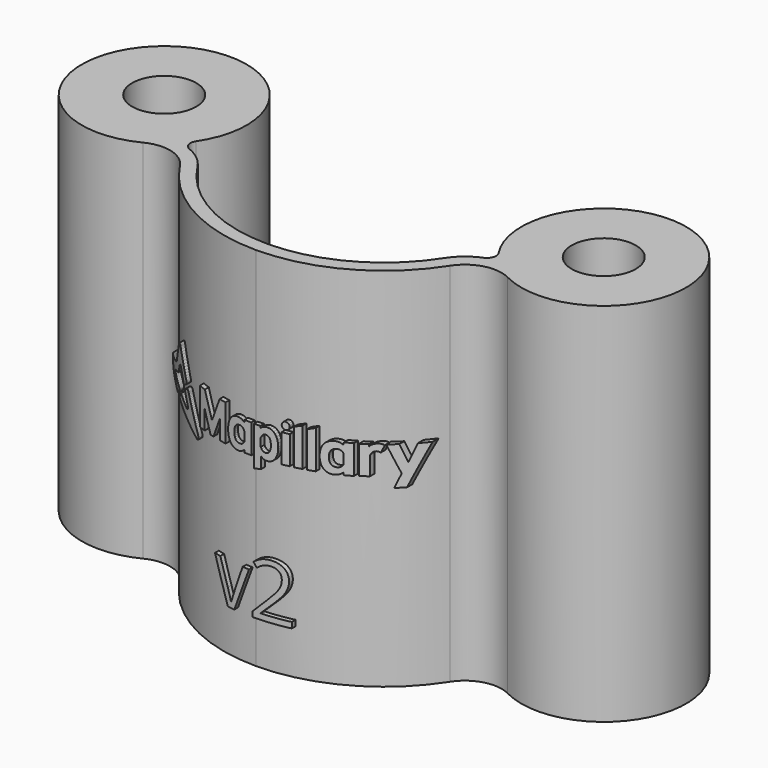
from build123d import *

# Parameters (mm, degrees)
F0_R         = 3.5
F1_DEPTH     = 40
F2_R         = 1
F4_W         = 0.766563
F4_H         = 3.09612
F4_TEXT_SIZE = 8.333333
F5_DEPTH     = 25
F6_W         = 87.868996
F6_H         = 45.529967
F7_DEPTH     = 60


# Not quite as in the source:
# - Text() gives the source's letters only with a copy of the font that has no kerning and outlines rounded to 1/6400 em; it was checked with that copy


with BuildPart() as f1:
    # F0 (on Top) → F1 (new body)
    with BuildSketch(Plane.XY):
        with BuildLine():
            ThreePointArc((-13.476744, -8.624231), (-15.168201, -6.941285), (-17.413215, -6.133047))
            ThreePointArc((-17.413215, -6.133047), (-29.41554, 7.188318), (-19.921875, -8.023023))
            ThreePointArc((-19.921875, -8.023023), (-17.059302, -7.729103), (-14.740189, -9.432753))
            ThreePointArc((-14.740189, -9.432753), (-8.401691, -15.351273), (0, -17.5))
            ThreePointArc((0, -17.5), (8.401691, -15.351273), (14.740189, -9.432753))
            ThreePointArc((14.740189, -9.432753), (17.059302, -7.729103), (19.921875, -8.023023))
            ThreePointArc((19.921875, -8.023023), (29.41554, 7.188318), (17.413215, -6.133047))
            ThreePointArc((17.413215, -6.133047), (15.168201, -6.941285), (13.476744, -8.624231))
            ThreePointArc((13.476744, -8.624231), (7.681546, -14.03545), (0, -16))
            ThreePointArc((0, -16), (-7.681546, -14.03545), (-13.476744, -8.624231))
        make_face()
        with Locations((-24, 0)):
            Circle(F0_R, mode=Mode.SUBTRACT)
        with Locations((24, 0)):
            Circle(F0_R, mode=Mode.SUBTRACT)
    extrude(amount=F1_DEPTH)

    # F2
    f2_edges = [f1.edges().sort_by_distance(p)[0] for p in [
        (-17.413215, -6.133047, 20),
        (17.413215, -6.133047, 20),
    ]]
    fillet(f2_edges, radius=F2_R)

    # F4 (on offset) → F5 (join)
    with BuildSketch(Plane.XZ.offset(25)):
        Polygon((-10.73702, 20.972938), (-10.658014, 20.9132), (-10.637207, 20.902077), (-10.599738, 20.881931), (-10.546861, 20.853384), (-10.479554, 20.816981), (-10.399024, 20.773344), (-10.306352, 20.723018), (-10.202674, 20.666702), (-10.089023, 20.605097), (-9.966599, 20.538592), (-9.836497, 20.467886), (-9.699768, 20.393602), (-9.557594, 20.316362), (-9.411072, 20.236711), (-9.261307, 20.155271), (-9.109379, 20.072742), (-8.956447, 19.989513), (-8.803601, 19.90644), (-8.651977, 19.823911), (-8.502616, 19.742782), (-8.356739, 19.663364), (-8.215367, 19.586436), (-8.079641, 19.512541), (-7.950683, 19.44238), (-7.829612, 19.376419), (-7.717486, 19.315436), (-7.61548, 19.259898), (-7.524667, 19.210505), (-7.446214, 19.167724), (-7.381139, 19.132332), (-7.330665, 19.104719), (-7.29581, 19.085739), (-7.27771, 19.075705), (-7.203309, 19.04887), (-7.131647, 19.048481), (-7.066658, 19.070416), (-7.012178, 19.110786), (-6.972096, 19.165779), (-6.950231, 19.231118), (-6.950519, 19.303302), (-6.976771, 19.377974), (-6.986649, 19.396331), (-7.005551, 19.431957), (-7.032939, 19.483761), (-7.068222, 19.550266), (-7.110754, 19.630539), (-7.159921, 19.723569), (-7.215171, 19.828033), (-7.275851, 19.942765), (-7.341384, 20.066675), (-7.411141, 20.198597), (-7.484577, 20.33752), (-7.561, 20.482042), (-7.639873, 20.631232), (-7.720566, 20.783767), (-7.802473, 20.938713), (-7.884978, 21.094748), (-7.967515, 21.250861), (-8.049469, 21.405729), (-8.130201, 21.558264), (-8.209113, 21.707376), (-8.285621, 21.851899), (-8.359135, 21.990744), (-8.429071, 22.122666), (-8.494728, 22.246576), (-8.55554, 22.36123), (-8.611, 22.465538), (-8.66037, 22.55849), (-8.703073, 22.638763), (-8.738566, 22.705191), (-8.766249, 22.75684), (-8.785408, 22.792231), (-8.795535, 22.810511), (-8.852722, 22.874605), (-8.930203, 22.913886), (-9.016878, 22.922131), (-9.101491, 22.89304), (-9.181671, 22.843491), (-9.261346, 22.795032), (-9.33405, 22.75225), (-9.393306, 22.719581), (-9.473525, 22.659998), (-9.512899, 22.589293), (-9.515396, 22.509719), (-9.484882, 22.423301), (-9.45656, 22.368697), (-9.422468, 22.303203), (-9.383599, 22.229074), (-9.340849, 22.147945), (-9.295236, 22.061605), (-9.24771, 21.97192), (-9.199313, 21.880679), (-9.150908, 21.789672), (-9.103514, 21.700764), (-9.058064, 21.615902), (-9.015571, 21.536562), (-8.977006, 21.464845), (-8.943317, 21.402384), (-8.915471, 21.351202), (-8.894414, 21.312855), (-8.881121, 21.289286), (-8.857778, 21.223714), (-8.860314, 21.159465), (-8.884116, 21.100115), (-8.924455, 21.049322), (-8.976702, 21.010819), (-9.036207, 20.987951), (-9.098193, 20.984606), (-9.158079, 21.004285), (-9.180746, 21.016808), (-9.222562, 21.039755), (-9.280877, 21.071491), (-9.352913, 21.110694), (-9.435932, 21.155731), (-9.527251, 21.205357), (-9.624061, 21.257939), (-9.723694, 21.312077), (-9.823414, 21.366293), (-9.920442, 21.41903), (-10.012095, 21.469045), (-10.095612, 21.514627), (-10.168278, 21.554375), (-10.227362, 21.586966), (-10.270113, 21.61069), (-10.293782, 21.624225), (-10.355566, 21.646316), (-10.428994, 21.643204), (-10.505285, 21.605323), (-10.575594, 21.523183), (-10.624256, 21.442054), (-10.673042, 21.359837), (-10.716718, 21.285008), (-10.750103, 21.225737), (-10.783309, 21.13294), (-10.778883, 21.047378), align=None)
        Polygon((-14.0382, 22.762674), (-13.984522, 22.721137), (-13.971987, 22.714292), (-13.946161, 22.700213), (-13.907969, 22.679289), (-13.858215, 22.652142), (-13.797826, 22.619162), (-13.727689, 22.58097), (-13.648688, 22.537877), (-13.561629, 22.490273), (-13.467476, 22.439014), (-13.367041, 22.384254), (-13.261201, 22.326538), (-13.150887, 22.266488), (-13.036949, 22.204339), (-12.920257, 22.140712), (-12.801683, 22.076073), (-12.682121, 22.010968), (-12.562442, 21.945784), (-12.443526, 21.88099), (-12.326251, 21.817052), (-12.211465, 21.754513), (-12.100054, 21.693919), (-11.992907, 21.635426), (-11.890947, 21.579888), (-11.794938, 21.527617), (-11.705899, 21.47908), (-11.624583, 21.43482), (-11.55191, 21.395306), (-11.48878, 21.360925), (-11.436073, 21.332223), (-11.394591, 21.309588), (-11.365298, 21.293642), (-11.34901, 21.284775), (-11.270977, 21.259495), (-11.193076, 21.264006), (-11.122557, 21.296131), (-11.066855, 21.353692), (-11.030102, 21.412341), (-10.977894, 21.498992), (-10.918054, 21.600034), (-10.85834, 21.701464), (-10.835938, 21.778237), (-10.848002, 21.857733), (-10.88831, 21.928127), (-10.950677, 21.977365), (-10.977816, 21.991288), (-11.021787, 22.014623), (-11.080149, 22.046048), (-11.150411, 22.084085), (-11.230039, 22.12741), (-11.316558, 22.174625), (-11.40741, 22.224252), (-11.500214, 22.274967), (-11.592373, 22.325527), (-11.681428, 22.374297), (-11.764898, 22.419957), (-11.840224, 22.461104), (-11.904956, 22.496496), (-11.956566, 22.524654), (-11.992565, 22.5441), (-12.010463, 22.553512), (-12.074603, 22.597071), (-12.114942, 22.649731), (-12.133891, 22.707758), (-12.133821, 22.767341), (-12.117019, 22.82459), (-12.085828, 22.875772), (-12.042658, 22.916997), (-11.989819, 22.944455), (-11.903696, 22.973857), (-11.807096, 23.006682), (-11.703962, 23.041841), (-11.59795, 23.077933), (-11.492949, 23.113636), (-11.392732, 23.147783), (-11.301071, 23.179052), (-11.221778, 23.206043), (-11.166411, 23.233034), (-11.117913, 23.272704), (-11.079052, 23.322175), (-11.052427, 23.378568), (-11.024238, 23.46382), (-10.9917, 23.56175), (-10.956542, 23.66777), (-10.920333, 23.776979), (-10.884724, 23.884476), (-10.851253, 23.985518), (-10.821548, 24.07497), (-10.79724, 24.148165), (-10.761537, 24.222837), (-10.715069, 24.272619), (-10.661437, 24.300077), (-10.604258, 24.307233), (-10.547117, 24.296732), (-10.493602, 24.270675), (-10.447351, 24.231705), (-10.411944, 24.181923), (-10.34505, 24.056691), (-10.263734, 23.9061), (-10.174407, 23.741198), (-10.083539, 23.573807), (-9.997534, 23.414816), (-9.922923, 23.275893), (-9.866117, 23.168318), (-9.833502, 23.103524), (-9.787586, 23.036007), (-9.726184, 22.995715), (-9.653852, 22.988014), (-9.575197, 23.018506), (-9.512946, 23.056931), (-9.425719, 23.109591), (-9.33013, 23.167696), (-9.242568, 23.222378), (-9.178591, 23.28056), (-9.142554, 23.351422), (-9.134658, 23.429361), (-9.154913, 23.508623), (-9.177829, 23.554672), (-9.226833, 23.648713), (-9.298145, 23.784135), (-9.388025, 23.95386), (-9.492823, 24.150887), (-9.608698, 24.368449), (-9.731916, 24.599468), (-9.858743, 24.836865), (-9.985461, 25.074029), (-10.108306, 25.303726), (-10.223512, 25.51911), (-10.327377, 25.713415), (-10.416121, 25.879329), (-10.485963, 26.010161), (-10.533272, 26.098835), (-10.554165, 26.138583), (-10.596821, 26.201899), (-10.649116, 26.247092), (-10.707314, 26.27385), (-10.767737, 26.282406), (-10.826689, 26.27245), (-10.880454, 26.244058), (-10.925358, 26.197077), (-10.957678, 26.131427), (-10.973258, 26.084601), (-10.998118, 26.009695), (-11.03102, 25.910287), (-11.070869, 25.790188), (-11.116528, 25.652588), (-11.166746, 25.500986), (-11.220386, 25.339118), (-11.276344, 25.170482), (-11.333352, 24.998423), (-11.390321, 24.826676), (-11.44603, 24.658506), (-11.499366, 24.497649), (-11.549133, 24.347603), (-11.594146, 24.211792), (-11.633311, 24.093716), (-11.665342, 23.99703), (-11.691765, 23.940248), (-11.729701, 23.891633), (-11.777515, 23.853052), (-11.833558, 23.826061), (-11.927537, 23.793625), (-12.041989, 23.754188), (-12.173475, 23.708918), (-12.318698, 23.658902), (-12.474328, 23.605465), (-12.636928, 23.549538), (-12.803208, 23.492522), (-12.969774, 23.435506), (-13.133246, 23.379657), (-13.290362, 23.326142), (-13.437646, 23.276127), (-13.5718, 23.230778), (-13.689497, 23.191342), (-13.787276, 23.158828), (-13.861886, 23.134637), (-13.90991, 23.119625), (-13.980807, 23.088589), (-14.034487, 23.044408), (-14.070779, 22.991048), (-14.089516, 22.932243), (-14.090445, 22.872116), (-14.073438, 22.814167), align=None)
        Polygon((-3.111755, 20.471153), (-3.111755, 24.431454), (-3.895196, 24.431454), (-4.935948, 21.936217), (-5.976778, 24.431454), (-6.760243, 24.431454), (-6.760243, 20.471153), (-5.99918, 20.471153), (-5.99918, 22.531343), (-5.14301, 20.471153), (-4.728887, 20.471153), (-3.872717, 22.531343), (-3.872717, 20.471153), align=None)
        Polygon((0.875461, 23.567273), (0.20955, 23.567273), (0.20955, 19.275999), (0.970513, 19.442924), (0.970513, 20.677203), (1.059342, 20.566983), (1.191575, 20.476909), (1.274649, 20.441906), (1.369934, 20.416782), (1.47751, 20.401769), (1.597375, 20.396713), (1.82326, 20.422538), (2.031022, 20.499777), (2.216381, 20.628588), (2.375217, 20.808736), (2.505116, 21.03921), (2.604524, 21.318144), (2.641238, 21.475968), (2.667452, 21.645771), (2.683164, 21.827864), (2.688453, 22.022091), (2.666752, 22.389854), (2.601724, 22.714603), (2.499671, 22.993615), (2.366738, 23.223933), (2.205103, 23.404937), (2.016943, 23.535848), (1.808559, 23.615265), (1.586096, 23.641712), (1.355233, 23.617443), (1.144049, 23.544404), (1.051642, 23.4933), (0.976113, 23.43714), (0.917386, 23.375924), (0.875461, 23.309729), align=None)
        Polygon((1.536859, 21.14873), (1.407115, 21.13504), (1.265004, 21.161487), (1.130126, 21.240905), (1.011816, 21.373215), (0.920186, 21.558497), (0.920186, 22.439869), (1.001938, 22.610839), (1.113247, 22.757462), (1.180219, 22.816345), (1.255203, 22.858348), (1.338276, 22.88355), (1.429439, 22.891951), (1.550549, 22.878027), (1.656724, 22.836257), (1.74781, 22.766407), (1.823883, 22.668788), (1.883854, 22.544333), (1.926713, 22.394054), (1.95246, 22.218029), (1.961016, 22.016335), (1.952304, 21.809818), (1.926402, 21.630759), (1.883076, 21.479313), (1.822482, 21.355403), (1.744621, 21.25895), (1.649413, 21.190112), align=None, mode=Mode.SUBTRACT)
        with Locations((3.401928, 22.019213)):
            Rectangle(F4_W, F4_H)
        Polygon((3.045171, 24.408508), (3.018647, 24.254029), (3.045171, 24.105928), (3.1249, 23.982251), (3.181994, 23.933403), (3.24671, 23.898555), (3.319049, 23.877554), (3.399089, 23.870631), (3.545401, 23.898555), (3.670634, 23.982251), (3.756585, 24.105928), (3.78521, 24.254029), (3.756585, 24.408508), (3.670634, 24.540275), (3.545401, 24.630349), (3.399089, 24.660373), (3.319049, 24.652906), (3.24671, 24.630349), (3.181994, 24.592857), (3.1249, 24.540275), align=None)
        Polygon((4.943649, 24.643183), (4.182609, 24.379884), (4.182609, 20.471153), (4.943649, 20.471153), align=None)
        Polygon((6.101933, 24.643183), (5.340893, 24.379884), (5.340893, 20.471153), (6.101933, 20.471153), align=None)
        Polygon((10.23157, 23.355544), (10.23157, 23.567273), (9.515334, 23.567273), (9.515334, 20.471153), (10.276296, 20.471153), (10.276296, 22.468494), (10.359603, 22.66241), (10.463756, 22.797521), (10.584788, 22.876938), (10.718421, 22.903463), (10.879279, 22.87196), (11.026213, 22.77753), (11.300402, 23.469965), (11.219896, 23.548682), (11.112943, 23.601653), (10.990433, 23.631678), (10.863878, 23.641712), (10.672295, 23.622422), (10.488958, 23.564472), (10.335101, 23.473621), align=None)
        Polygon((8.196037, 20.573283), (8.354095, 20.69696), (8.354095, 20.433816), (9.12968, 20.433816), (9.12968, 23.588819), (8.354095, 23.588819), (8.354095, 23.33921), (8.204594, 23.458608), (8.03938, 23.550627), (7.858843, 23.609743), (7.662905, 23.630667), (7.505081, 23.622422), (7.358847, 23.597842), (7.22428, 23.557861), (7.100759, 23.503567), (6.988438, 23.435273), (6.887008, 23.354144), (6.796156, 23.261037), (6.715727, 23.156417), (6.645566, 23.041452), (6.585361, 22.916686), (6.535035, 22.783209), (6.494276, 22.641641), (6.463084, 22.492918), (6.440916, 22.337661), (6.427848, 22.176881), (6.423492, 22.011279), (6.427848, 21.845754), (6.440916, 21.684896), (6.463084, 21.529639), (6.494276, 21.380916), (6.535035, 21.239349), (6.585361, 21.105871), (6.645566, 20.981183), (6.715727, 20.866141), (6.796156, 20.761676), (6.887008, 20.668413), (6.988438, 20.587284), (7.100759, 20.51899), (7.22428, 20.464697), (7.358847, 20.424716), (7.505081, 20.400214), (7.662905, 20.391735), (7.848809, 20.414137), (8.02709, 20.476753), align=None)
        Polygon((8.354095, 22.498596), (8.354095, 21.478768), (8.26721, 21.333468), (8.152245, 21.222936), (8.009044, 21.151997), (7.837219, 21.125084), (7.674572, 21.14033), (7.537672, 21.189723), (7.425119, 21.269762), (7.335667, 21.376716), (7.267606, 21.507082), (7.219846, 21.657283), (7.190988, 21.823741), (7.179554, 22.002722), (7.184766, 22.182093), (7.207945, 22.349406), (7.250493, 22.501241), (7.313965, 22.634019), (7.399683, 22.744083), (7.509437, 22.828012), (7.644548, 22.88215), (7.806572, 22.903074), (7.895013, 22.897396), (7.978786, 22.877172), (8.057193, 22.843491), (8.129999, 22.796976), (8.196426, 22.73856), (8.256398, 22.668788), (8.309058, 22.588593), align=None, mode=Mode.SUBTRACT)
        Polygon((-1.024417, 20.573283), (-0.866282, 20.69696), (-0.866282, 20.433816), (-0.090696, 20.433816), (-0.090696, 23.588819), (-0.866282, 23.588819), (-0.866282, 23.33921), (-1.015861, 23.458608), (-1.180919, 23.550627), (-1.361611, 23.609743), (-1.557472, 23.630667), (-1.715296, 23.622422), (-1.861452, 23.597842), (-1.996174, 23.557861), (-2.11954, 23.503567), (-2.231938, 23.435273), (-2.333446, 23.354144), (-2.424221, 23.261037), (-2.504727, 23.156417), (-2.574811, 23.041452), (-2.635016, 22.916686), (-2.685342, 22.783209), (-2.726023, 22.641641), (-2.75737, 22.492918), (-2.779461, 22.337661), (-2.792528, 22.176881), (-2.796807, 22.011279), (-2.792528, 21.845754), (-2.779461, 21.684896), (-2.75737, 21.529639), (-2.726023, 21.380916), (-2.685342, 21.239349), (-2.635016, 21.105871), (-2.574811, 20.981183), (-2.504727, 20.866141), (-2.424221, 20.761676), (-2.333446, 20.668413), (-2.231938, 20.587284), (-2.11954, 20.51899), (-1.996174, 20.464697), (-1.861452, 20.424716), (-1.715296, 20.400214), (-1.557472, 20.391735), (-1.371646, 20.414137), (-1.193364, 20.476753), align=None)
        Polygon((-0.866282, 22.498596), (-0.866282, 21.478768), (-0.953089, 21.333468), (-1.068054, 21.222936), (-1.21141, 21.151997), (-1.383158, 21.125084), (-1.545804, 21.14033), (-1.682704, 21.189723), (-1.795258, 21.269762), (-1.884788, 21.376716), (-1.952771, 21.507082), (-2.00053, 21.657283), (-2.02931, 21.823741), (-2.040823, 22.002722), (-2.035611, 22.182093), (-2.012354, 22.349406), (-1.969961, 22.501241), (-1.906412, 22.634019), (-1.820616, 22.744083), (-1.71094, 22.828012), (-1.575829, 22.88215), (-1.413805, 22.903074), (-1.325364, 22.897396), (-1.241668, 22.877172), (-1.163106, 22.843491), (-1.090456, 22.796976), (-1.023873, 22.73856), (-0.964057, 22.668788), (-0.911319, 22.588593), align=None, mode=Mode.SUBTRACT)
        Polygon((11.91023, 19.372374), (12.704951, 19.372374), (14.182149, 23.567273), (13.359582, 23.567273), (12.794402, 21.770226), (12.229223, 23.567273), (11.389854, 23.567273), (12.38588, 20.74013), align=None)
        with Locations((-4.516276, 4.92436)):
            Text('v2', F4_TEXT_SIZE, font='Open Sans', text_align=(TextAlign.LEFT, TextAlign.BOTTOM))
    extrude(amount=-F5_DEPTH)

    # F6 (on Top) → F7 (cut)
    with BuildSketch(Plane.XY):
        with Locations((0, -2.235017)):
            Rectangle(F6_W, F6_H)
        with BuildLine():
            ThreePointArc((15.161337, -9.70226), (0, -18), (-15.161337, -9.70226))
            ThreePointArc((-15.161337, -9.70226), (-17.190561, -8.211566), (-19.695312, -8.468746))
            Line((-19.695312, -8.468746), (-19.921875, -8.023023))
            ThreePointArc((-19.921875, -8.023023), (-29.974356, 6.731053), (-16.517737, -5.001574))
            ThreePointArc((-16.517737, -5.001574), (-16.641776, -5.852616), (-16.059144, -6.485229))
            ThreePointArc((-16.059144, -6.485229), (-14.600957, -7.353128), (-13.476744, -8.624231))
            ThreePointArc((-13.476744, -8.624231), (0, -16), (13.476744, -8.624231))
            ThreePointArc((13.476744, -8.624231), (14.600957, -7.353128), (16.059144, -6.485229))
            ThreePointArc((16.059144, -6.485229), (16.641776, -5.852616), (16.517737, -5.001574))
            ThreePointArc((16.517737, -5.001574), (29.974356, 6.731053), (19.921875, -8.023023))
            Line((19.921875, -8.023023), (19.695312, -8.468746))
            ThreePointArc((19.695312, -8.468746), (17.190561, -8.211566), (15.161337, -9.70226))
        make_face(mode=Mode.SUBTRACT)
    extrude(amount=F7_DEPTH, mode=Mode.SUBTRACT)


solid = f1.part
